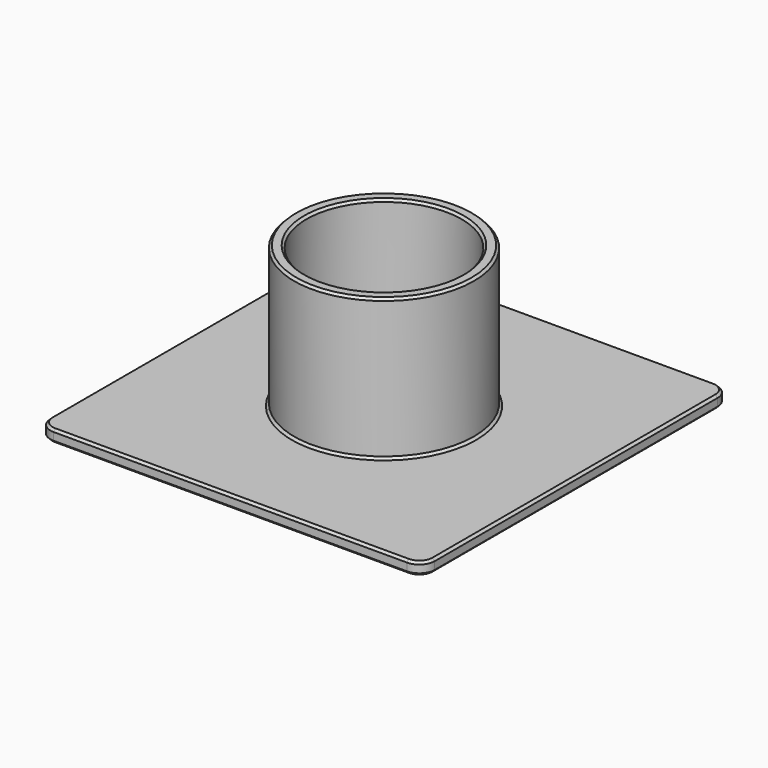
from build123d import *

# Parameters (mm, degrees)
F1_W     = 50
F1_H     = 50
F1_R     = 11.7
F1_R_2   = 10.1
F2_DEPTH = 1.6
F5_DEPTH = 20
F3_R     = 2
F4_SIZE  = 0.3


with BuildPart() as f2:
    # F1 (on Top) → F2 (new body)
    with BuildSketch(Plane.XY):
        Rectangle(F1_W, F1_H)
        Circle(F1_R, mode=Mode.SUBTRACT)
        Circle(F1_R)
        Circle(F1_R_2, mode=Mode.SUBTRACT)
        Circle(F1_R_2)
    extrude(amount=F2_DEPTH)

    # F1 (on Top) → F5 (join)
    with BuildSketch(Plane.XY):
        Circle(F1_R)
        Circle(F1_R_2, mode=Mode.SUBTRACT)
    extrude(amount=F5_DEPTH)

    # F3
    f3_edges = [f2.edges().sort_by_distance(p)[0] for p in [
        (25, 25, 0.8),
        (25, -25, 0.8),
        (-25, -25, 0.8),
        (-25, 25, 0.8),
    ]]
    fillet(f3_edges, radius=F3_R)

    # F4
    f4_edges = [f2.edges().sort_by_distance(p)[0] for p in [
        (0, 25, 1.6),
        (24.414214, 24.414214, 1.6),
        (-24.414214, 24.414214, 1.6),
        (25, 0, 1.6),
        (-25, 0, 1.6),
        (24.414214, -24.414214, 1.6),
        (-24.414214, -24.414214, 1.6),
        (0, -25, 1.6),
        (-11.7, 0, 1.6),
        (0, 25, 0),
        (24.414214, 24.414214, 0),
        (-24.414214, 24.414214, 0),
        (25, 0, 0),
        (-25, 0, 0),
        (24.414214, -24.414214, 0),
        (-24.414214, -24.414214, 0),
        (0, -25, 0),
        (-10.1, 0, 20),
        (-11.7, 0, 20),
        (-10.1, 0, 1.6),
    ]]
    chamfer(f4_edges, length=F4_SIZE)


solid = f2.part
